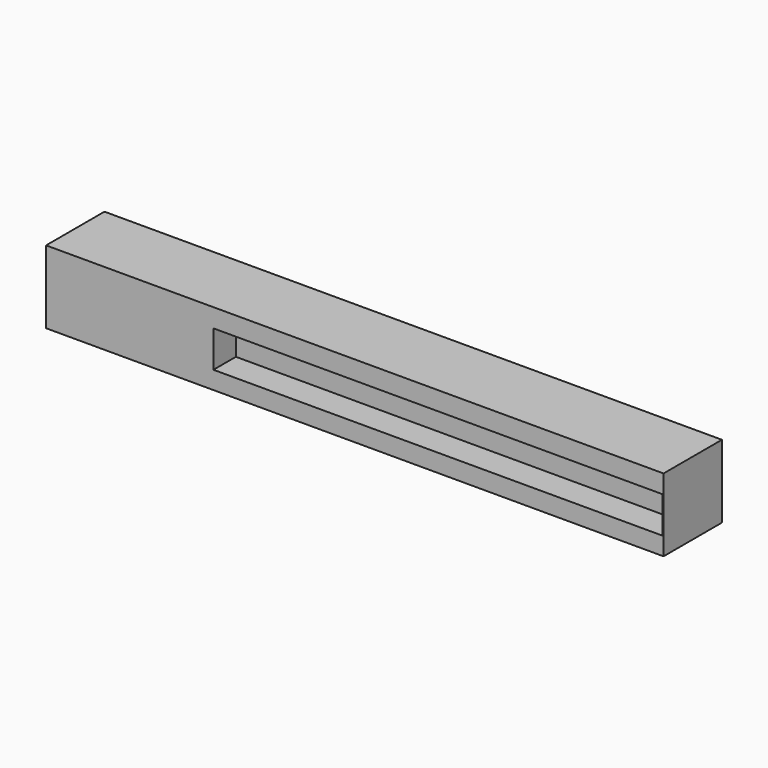
from build123d import *

# Parameters (mm, degrees)
F0_W     = 13
F0_H     = 13
F1_DEPTH = 110
F2_W     = 80
F2_H     = 6.5
F3_DEPTH = 5


# Not quite as in the source:
# - a pattern or mirror of a feature is missing from the dataset's text; its kind, count and spacing are read off the source's solid


with BuildPart() as f1:
    # F0 (on Right) → F1 (new body)
    with BuildSketch(Plane.YZ):
        Rectangle(F0_W, F0_H)
    extrude(amount=F1_DEPTH)

    # F2 (on face) → F3 (cut)
    with BuildSketch(Plane.XZ.offset(6.5)):
        with Locations((69.8135038838, -0.0667710053)):
            Rectangle(F2_W, F2_H)
    f3 = extrude(amount=-F3_DEPTH, mode=Mode.SUBTRACT)

    # F3_copies: F3 across plane
    add(f3.mirror(Plane.ZX), mode=Mode.SUBTRACT)


solid = f1.part
